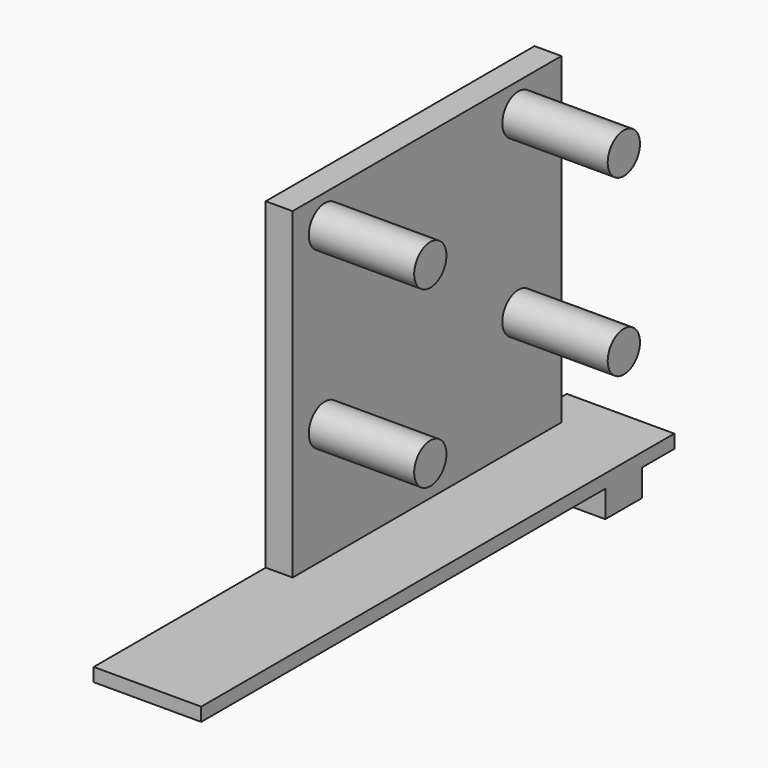
from build123d import *

# Parameters (mm, degrees)
F0_W     = 6
F0_H     = 3.4142509103
F0_W_2   = 2
F1_DEPTH = 2
F0_H_2   = 21.5857490897
F2_DEPTH = 1
F3_DEPTH = 25
F4_R     = 1.5
F5_DEPTH = 10


with BuildPart() as f1:
    # F0 (on Top) → F1 (new body)
    with BuildSketch(Plane.XY):
        with Locations((5.1546765715, 36.1676104367)):
            Rectangle(F0_W, F0_H)
        with Locations((1.1546765715, 36.1676104367)):
            Rectangle(F0_W_2, F0_H)
    extrude(amount=-F1_DEPTH)

    # F0 (on Top) → F2 (join)
    with BuildSketch(Plane.XY):
        Polygon((2.1546765715, 12.8747358918), (0.1546765715, 12.8747358918), (0.1546765715, -3.1252641082), (8.1546765715, -3.1252641082), (8.1546765715, 34.4604849815), (2.1546765715, 34.4604849815), align=None)
        with Locations((1.1546765715, 36.1676104367)):
            Rectangle(F0_W_2, F0_H)
        with Locations((5.1546765715, 36.1676104367)):
            Rectangle(F0_W, F0_H)
        Polygon((4, 40.8747358918), (0.1546765715, 40.8747358918), (0.1546765715, 37.8747358918), (2.1546765715, 37.8747358918), (8.1546765715, 37.8747358918), (8.1546765715, 40.8747358918), align=None)
        with Locations((1.1546765715, 23.6676104367)):
            Rectangle(F0_W_2, F0_H_2)
    extrude(amount=F2_DEPTH)


with BuildPart() as f3:
    # F0 (on Top) → F3 (new body)
    with BuildSketch(Plane.XY):
        with Locations((1.1546765715, 36.1676104367)):
            Rectangle(F0_W_2, F0_H)
        with Locations((1.1546765715, 23.6676104367)):
            Rectangle(F0_W_2, F0_H_2)
    extrude(amount=F3_DEPTH)


with BuildPart() as f5:
    # F4 (on Right) → F5 (new body)
    with BuildSketch(Plane.YZ):
        with Locations((15.8747358918, 9.8151313141)):
            Circle(F4_R)
    extrude(amount=F5_DEPTH)


with BuildPart() as f5b:
    # F4 (on Right) → F5, piece 2 (new body)
    with BuildSketch(Plane.YZ):
        with Locations((15.8747358918, 22.8151313141)):
            Circle(F4_R)
    extrude(amount=F5_DEPTH)


with BuildPart() as f5c:
    # F4 (on Right) → F5, piece 3 (new body)
    with BuildSketch(Plane.YZ):
        with Locations((33.8747358918, 22.8151313141)):
            Circle(F4_R)
    extrude(amount=F5_DEPTH)


with BuildPart() as f5d:
    # F4 (on Right) → F5, piece 4 (new body)
    with BuildSketch(Plane.YZ):
        with Locations((33.8747358918, 9.8151313141)):
            Circle(F4_R)
    extrude(amount=F5_DEPTH)


solid = Compound([f1.part, f3.part, f5.part, f5b.part, f5c.part, f5d.part])
